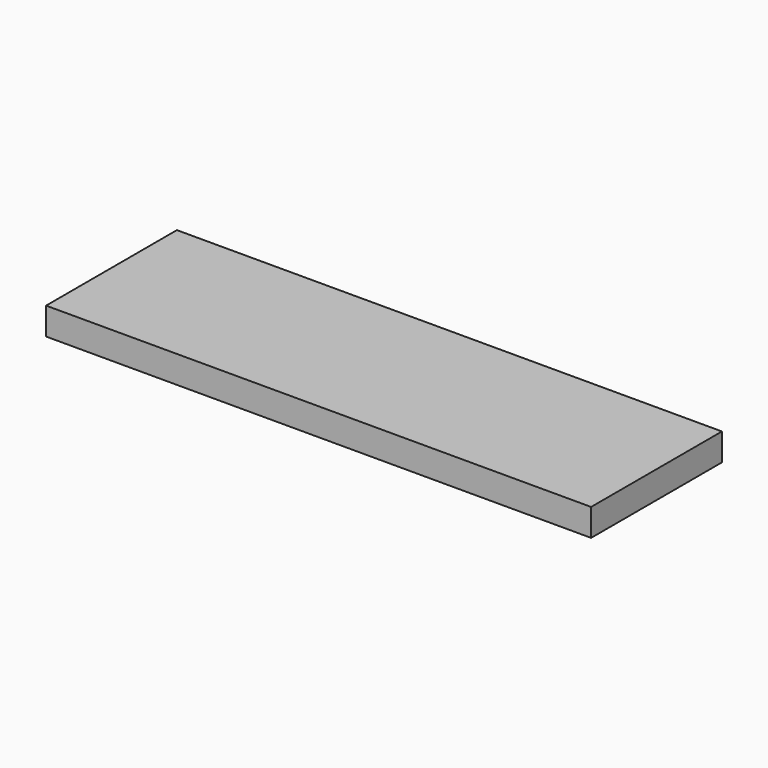
from build123d import *

# Parameters (mm, degrees)
F1_W     = 123.825
F1_H     = 31.75
F1_W_2   = 114.3
F1_H_2   = 25.4
F2_DEPTH = 6.35
F3_DEPTH = 6.35
F4_DEPTH = 6.35
F5_DEPTH = 6.35
F6_DEPTH = 6.35


# Not quite as in the source:
# - a variable given as a bare number and used for a length is read in inches; the dataset says mm whatever the document's units were


with BuildPart() as f2:
    # F1 (on Top) → F2 (new body)
    with BuildSketch(Plane.XY):
        with Locations((-1.5875, 0)):
            Rectangle(F1_W, F1_H)
        Rectangle(F1_W_2, F1_H_2, mode=Mode.SUBTRACT)
        Rectangle(F1_W_2, F1_H_2)
        Polygon((-63.5, -19.05), (63.5, -19.05), (63.5, 19.05), (-63.5, 19.05), (-63.5, 15.875), (60.325, 15.875), (60.325, -15.875), (-63.5, -15.875), align=None)
    extrude(amount=F2_DEPTH)


with BuildPart() as f3:
    # F1 (on Top) → F3 (new body)
    with BuildSketch(Plane.XY):
        with Locations((-1.5875, 0)):
            Rectangle(F1_W, F1_H)
        Rectangle(F1_W_2, F1_H_2, mode=Mode.SUBTRACT)
        Polygon((-63.5, -19.05), (63.5, -19.05), (63.5, 19.05), (-63.5, 19.05), (-63.5, 15.875), (60.325, 15.875), (60.325, -15.875), (-63.5, -15.875), align=None)
    extrude(amount=F3_DEPTH)


with BuildPart() as f4:
    # F1 (on Top) → F4 (new body)
    with BuildSketch(Plane.XY):
        Polygon((-63.5, -19.05), (63.5, -19.05), (63.5, 19.05), (-63.5, 19.05), (-63.5, 15.875), (60.325, 15.875), (60.325, -15.875), (-63.5, -15.875), align=None)
    extrude(amount=F4_DEPTH)


with BuildPart() as f5:
    # F1 (on Top) → F5 (new body)
    with BuildSketch(Plane.XY):
        with Locations((-1.5875, 0)):
            Rectangle(F1_W, F1_H)
        Rectangle(F1_W_2, F1_H_2, mode=Mode.SUBTRACT)
        Rectangle(F1_W_2, F1_H_2)
    extrude(amount=F5_DEPTH)


with BuildPart() as f6:
    # F1 (on Top) → F6 (new body)
    with BuildSketch(Plane.XY):
        with Locations((-1.5875, 0)):
            Rectangle(F1_W, F1_H)
        Rectangle(F1_W_2, F1_H_2, mode=Mode.SUBTRACT)
        Rectangle(F1_W_2, F1_H_2)
        Polygon((-63.5, -19.05), (63.5, -19.05), (63.5, 19.05), (-63.5, 19.05), (-63.5, 15.875), (60.325, 15.875), (60.325, -15.875), (-63.5, -15.875), align=None)
    extrude(amount=F6_DEPTH)


solid = Compound([f2.part, f3.part, f4.part, f5.part, f6.part])
